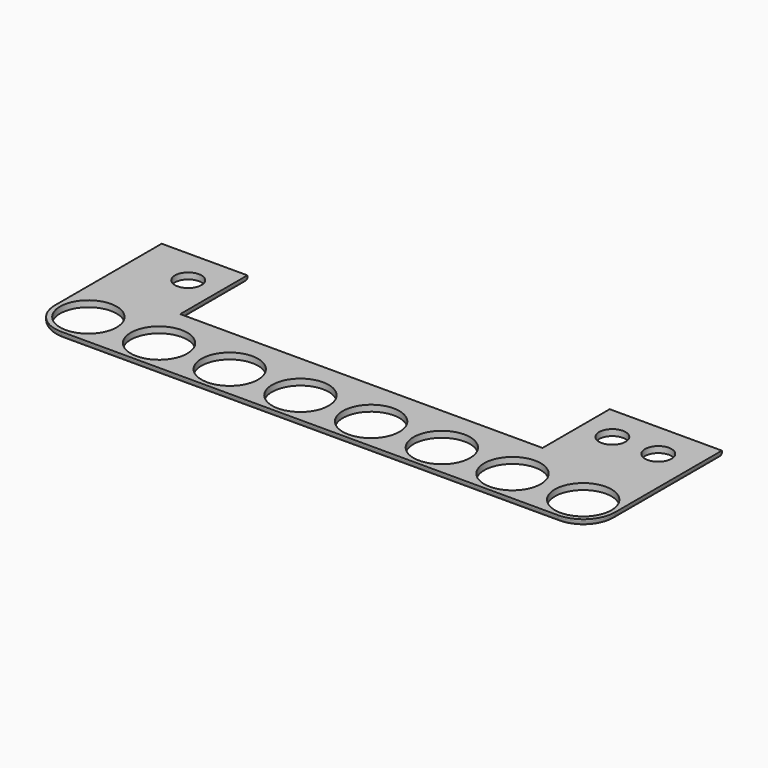
from build123d import *

# Parameters (mm, degrees)
F0_R        = 3.2
F0_R_2      = 1.5
F1_DEPTH    = 0.7
F2_R        = 0.49999
F3_T1_DEPTH = 9.7
F3_T4_ANGLE = 90
F3_T6_ANGLE = 90


# Not quite as in the source:
# - a fillet or chamfer that OpenCascade refuses, or shapes differently, is made with other operations: its cross-section is extruded or revolved along the edge and cut away or added
# - a fillet or chamfer is up to 0.001 mm smaller than in the source, because OpenCascade refuses the exact size


with BuildPart() as f1:
    # F0 (on Top) → F1 (new body)
    with BuildSketch(Plane.XY):
        Polygon((-22, 18.7), (-31.7, 18.7), (-31.7, 0), (-18.3513443917, 0), (-10.3513443917, 0), (31.7, 0), (31.7, 18.7), (19, 18.7), (19, 9.2), (-22, 9.2), align=None)
        with Locations((-28, 3.7)):
            Circle(F0_R, mode=Mode.SUBTRACT)
        with Locations((-20, 3.7)):
            Circle(F0_R, mode=Mode.SUBTRACT)
        with Locations((-12, 3.7)):
            Circle(F0_R, mode=Mode.SUBTRACT)
        with Locations((-4, 3.7)):
            Circle(F0_R, mode=Mode.SUBTRACT)
        with Locations((4, 3.7)):
            Circle(F0_R, mode=Mode.SUBTRACT)
        with Locations((12, 3.7)):
            Circle(F0_R, mode=Mode.SUBTRACT)
        with Locations((20, 3.7)):
            Circle(F0_R, mode=Mode.SUBTRACT)
        with Locations((28, 3.7)):
            Circle(F0_R, mode=Mode.SUBTRACT)
        with Locations((-25.5, 14.7)):
            Circle(F0_R_2, mode=Mode.SUBTRACT)
        with Locations((22.5, 14.7)):
            Circle(F0_R_2, mode=Mode.SUBTRACT)
        with Locations((27.7, 14.7)):
            Circle(F0_R_2, mode=Mode.SUBTRACT)
    extrude(amount=F1_DEPTH)

    # F2 (radius 0.5 in the source; OpenCascade refuses exactly that, so slightly less here)
    f2_edges = [f1.edges().sort_by_distance(p)[0] for p in [
        (-31.7, 9.35, 0),
        (0, 0, 0),
        (31.7, 9.35, 0),
        (25.35, 18.7, 0),
        (19, 13.95, 0),
        (-1.5, 9.2, 0),
        (-22, 13.95, 0),
        (-26.85, 18.7, 0),
    ]]
    fillet(f2_edges, radius=F2_R)

    # F3: fillet of radius 3.6 on 4 edges, made by hand

    # F3_s2 → F3_t1 (cut)
    with BuildSketch(Plane.XY):
        with BuildLine():
            ThreePointArc((-28.1, 0), (-30.6455844123, 1.0544155877), (-31.7, 3.6))
            Line((-31.7, 3.6), (-31.7, 0))
            Line((-31.7, 0), (-28.1, 0))
        make_face()
        with BuildLine():
            ThreePointArc((28.1, 0), (30.6455844123, 1.0544155877), (31.7, 3.6))
            Line((31.7, 3.6), (31.7, 0))
            Line((31.7, 0), (28.1, 0))
        make_face()
    extrude(amount=F3_T1_DEPTH, mode=Mode.SUBTRACT)

    # F3_s3 → F3_t4 (revolve, cut)
    with BuildSketch(Plane.YZ.offset(-28.1)):
        with BuildLine():
            ThreePointArc((0.49999, 0), (0.1464436805, 0.1464436805), (0, 0.49999))
            Line((0, 0.49999), (0, 0))
            Line((0, 0), (0.49999, 0))
        make_face()
    revolve(axis=Axis((-28.1, 3.6, 0), (0, 0, -1)), revolution_arc=F3_T4_ANGLE, mode=Mode.SUBTRACT)

    # F3_s5 → F3_t6 (revolve, cut)
    with BuildSketch(Plane.XZ.offset(-3.6)):
        with BuildLine():
            ThreePointArc((31.20001, 0), (31.5535563195, 0.1464436805), (31.7, 0.49999))
            Line((31.7, 0.49999), (31.7, 0))
            Line((31.7, 0), (31.20001, 0))
        make_face()
    revolve(axis=Axis((28.1, 3.6, 0), (0, 0, -1)), revolution_arc=F3_T6_ANGLE, mode=Mode.SUBTRACT)


solid = f1.part
